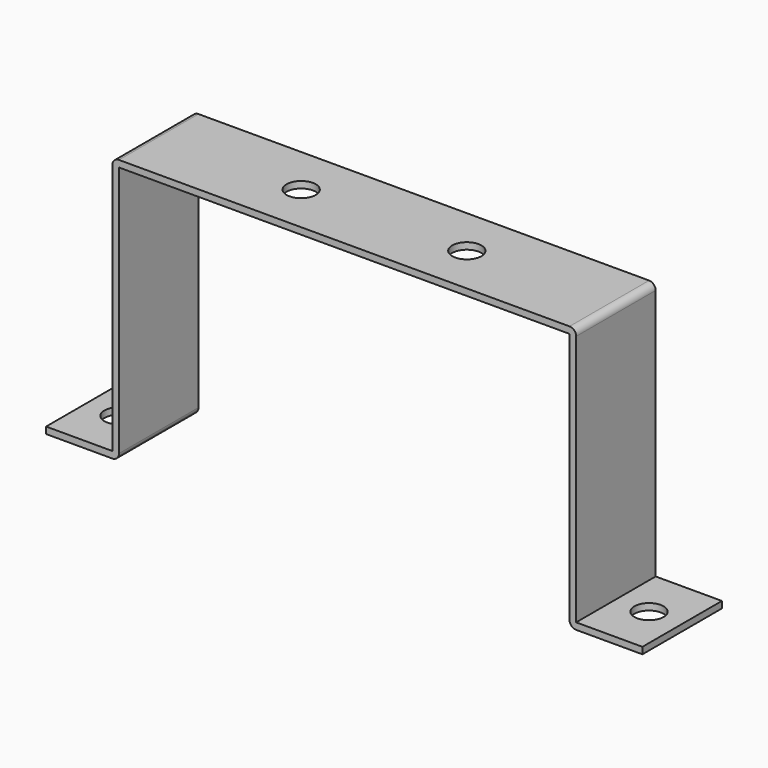
from build123d import *

# Parameters (mm, degrees)
F1_DEPTH = 30
F2_R     = 4.4
F3_R     = 4.4
F4_DEPTH = 25
F5_R     = 2
F6_R     = 2


# Not quite as in the source:
# - a feature names something its author has since deleted; it is built from what else it names


with BuildPart() as f1:
    # F0 (on Front) → F1 (new body)
    with BuildSketch(Plane.XZ):
        Polygon((90, -1), (90, 1), (70, 1), (70, 79), (-70, 79), (-70, 1), (-90, 1), (-90, -1), (-68, -1), (-68, 77), (68, 77), (68, -1), align=None)
    extrude(amount=F1_DEPTH)

    # F2 (on face) + F3 (on face) → F4 (cut)
    with BuildSketch(Plane.XY.offset(1)):
        with Locations((-80, -15)):
            Circle(F2_R)
        with Locations((80, -15)):
            Circle(F2_R)
    with BuildSketch(Plane.XY.offset(79)):
        with Locations((-25, -15)):
            Circle(F3_R)
        with Locations((25, -15)):
            Circle(F3_R)
    extrude(amount=-F4_DEPTH, mode=Mode.SUBTRACT)

    # F5
    f5_edges = [f1.edges().sort_by_distance(p)[0] for p in [
        (-70, -15, 79),
        (70, -15, 79),
    ]]
    fillet(f5_edges, radius=F5_R)

    # F6
    f6_edges = [f1.edges().sort_by_distance(p)[0] for p in [
        (68, -15, -1),
        (-68, -15, -1),
    ]]
    fillet(f6_edges, radius=F6_R)


solid = f1.part
